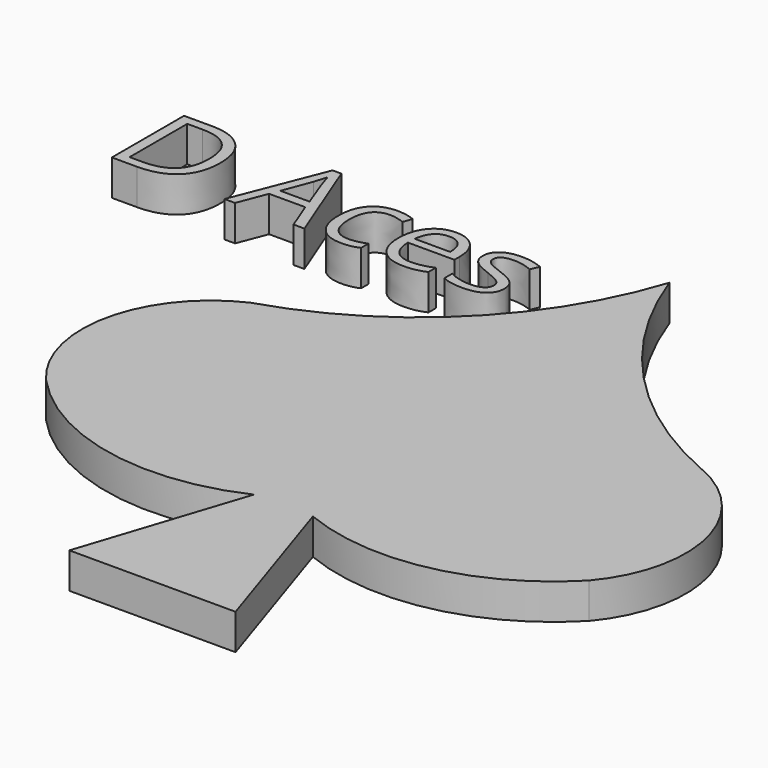
from build123d import *

# Parameters (mm, degrees)
F0_TEXT_SIZE = 10.6438761577
F1_DEPTH     = 3


# Not quite as in the source:
# - Text() gives the source's letters only with a copy of the font that has no kerning and outlines rounded to 1/6400 em; it was checked with that copy


with BuildPart() as f1:
    # F0 (on Top) → F1 (new body)
    with BuildSketch(Plane.XY):
        with BuildLine():
            Line((-2.4908845205, -15.4208163917), (-7.0029371418, -29.2009245604))
            Line((-7.0029371418, -29.2009245604), (6.9970628582, -29.2009245604))
            Line((6.9970628582, -29.2009245604), (2.4850102369, -15.4208163917))
            ThreePointArc((2.4850102369, -15.4208163917), (13.0685205169, -16.360261956), (22.3612855074, -11.2087799706))
            ThreePointArc((22.3612855074, -11.2087799706), (24.6278921181, -1.6844900086), (18.3013859417, 5.7871178777))
            ThreePointArc((18.3013859417, 5.7871178777), (7.1260467866, 13.6069647533), (0, 25.2369977534))
            ThreePointArc((0, 25.2369977534), (-7.5025163767, 13.1015138727), (-19.7523054455, 5.7871178777))
            ThreePointArc((-19.7523054455, 5.7871178777), (-25.8095597062, -1.8085439742), (-23.3559967133, -11.2087799706))
            ThreePointArc((-23.3559967133, -11.2087799706), (-13.6065541049, -16.6987289317), (-2.4908845205, -15.4208163917))
        make_face()
        with Locations((-40.828442201, 16.2521004677)):
            Text('D Aces', F0_TEXT_SIZE, font='Open Sans', text_align=(TextAlign.LEFT, TextAlign.BOTTOM))
    extrude(amount=F1_DEPTH)


solid = f1.part
